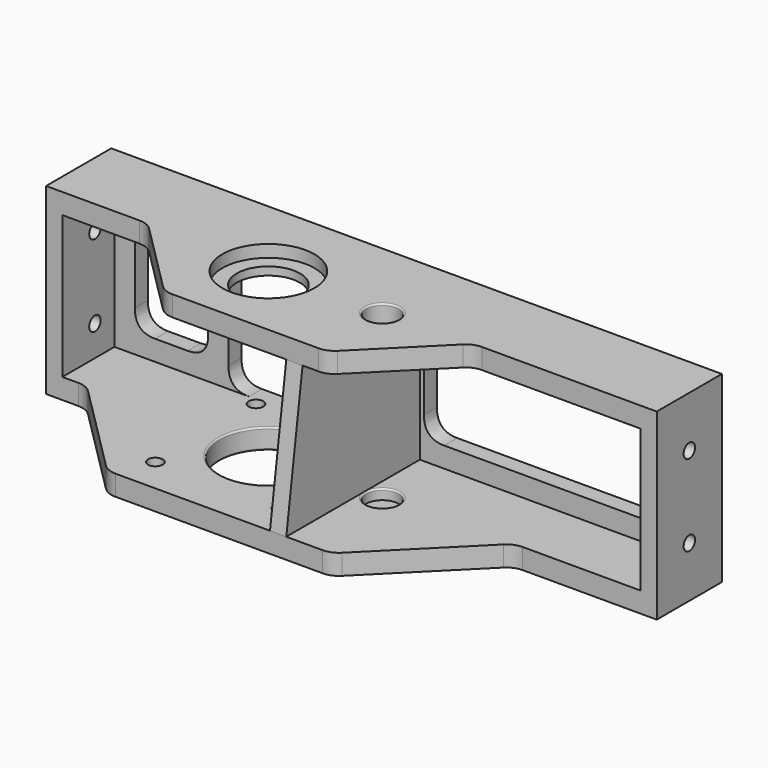
from build123d import *

# Parameters (mm, degrees)
F0_R         = 1.8
F0_R_2       = 12
F0_R_3       = 4
F1_DEPTH     = 5
F2_W         = 4
F2_H         = 20
F3_DEPTH     = 40
F4_R         = 12.5
F4_R_2       = 11.3
F4_R_3       = 7.75
F5_DEPTH     = 5
F6_DEPTH     = 50
F7_DEPTH     = 3
F8_R         = 5
F9_R         = 0.4
F10_DEPTH    = 2.5
F11_R        = 1.75
F12_DEPTH    = 150.001
F13_W        = 28
F13_H        = 4
F13_W_2      = 71
F14_DEPTH    = 40
F15_W        = 18
F15_H        = 25
F15_W_2      = 61
F16_DEPTH    = 25
F17_T1_DEPTH = 4
F19_DEPTH    = 41
F21_DEPTH    = 5


# Not quite as in the source:
# - a fillet or chamfer that OpenCascade refuses, or shapes differently, is made with other operations: its cross-section is extruded or revolved along the edge and cut away or added


with BuildPart() as f1:
    # F0 (on Top) → F1 (new body)
    with BuildSketch(Plane.XY):
        Polygon((75, 27), (-75, 27), (-75, 7), (-65, 7), (-40, -18), (15, -18), (40, 7), (75, 7), align=None)
        with Locations((-35, -9.44)):
            Circle(F0_R, mode=Mode.SUBTRACT)
        with Locations((-4.2, -9.44)):
            Circle(F0_R, mode=Mode.SUBTRACT)
        with Locations((-19.6, 6)):
            Circle(F0_R_2, mode=Mode.SUBTRACT)
        with Locations((-35, 21.44)):
            Circle(F0_R, mode=Mode.SUBTRACT)
        with Locations((-4.2, 21.44)):
            Circle(F0_R, mode=Mode.SUBTRACT)
        with Locations((8.4, 6)):
            Circle(F0_R_3, mode=Mode.SUBTRACT)
    extrude(amount=F1_DEPTH)

    # F2 (on face) → F3 (join)
    with BuildSketch(Plane.XY.offset(5)):
        with Locations((-73, 17)):
            Rectangle(F2_W, F2_H)
        with Locations((73, 17)):
            Rectangle(F2_W, F2_H)
    extrude(amount=F3_DEPTH)

    # F4 (on face) → F5 (join)
    with BuildSketch(Plane.XY.offset(45)):
        Polygon((71, 7), (71, 27), (-75, 27), (-75, 7), (-50, 7), (-30, -13), (10, -13), (30, 7), align=None)
        with Locations((-19.6, 6)):
            Circle(F4_R, mode=Mode.SUBTRACT)
        with Locations((-19.6, 6)):
            Circle(F4_R)
        with Locations((-19.6, 6)):
            Circle(F4_R_2, mode=Mode.SUBTRACT)
        with Locations((-19.6, 6)):
            Circle(F4_R_2)
        with Locations((-19.6, 6)):
            Circle(F4_R_3, mode=Mode.SUBTRACT)
    extrude(amount=-F5_DEPTH)

    # F0 (on Top) → F6 (cut)
    with BuildSketch(Plane.XY):
        with Locations((8.4, 6)):
            Circle(F0_R_3)
    extrude(amount=F6_DEPTH, mode=Mode.SUBTRACT)

    # F4 (on face) → F7 (cut)
    with BuildSketch(Plane.XY.offset(45)):
        with Locations((-19.6, 6)):
            Circle(F4_R_2)
        with Locations((-19.6, 6)):
            Circle(F4_R_3, mode=Mode.SUBTRACT)
    extrude(amount=-F7_DEPTH, mode=Mode.SUBTRACT)

    # F8
    f8_edges = [f1.edges().sort_by_distance(p)[0] for p in [
        (-65, 7, 2.5),
        (-40, -18, 2.5),
        (40, 7, 2.5),
        (15, -18, 2.5),
        (-50, 7, 42.5),
        (-30, -13, 42.5),
        (10, -13, 42.5),
        (30, 7, 42.5),
    ]]
    fillet(f8_edges, radius=F8_R)

    # F9
    f9_edges = [f1.edges().sort_by_distance(p)[0] for p in [
        (-31.6, 6, 5),
        (-31.6, 6, 0),
        (4.4, 6, 5),
        (4.4, 6, 45),
        (4.4, 6, 40),
    ]]
    fillet(f9_edges, radius=F9_R)

    # F0 (on Top) → F10 (join)
    with BuildSketch(Plane.XY):
        with Locations((8.4, 6)):
            Circle(F0_R_3)
    extrude(amount=F10_DEPTH)

    # F11 (on face) → F12 (cut, through all)
    with BuildSketch(Plane.YZ.offset(75)):
        with Locations((17, 32.5)):
            Circle(F11_R)
        with Locations((17, 12.5)):
            Circle(F11_R)
    extrude(amount=-F12_DEPTH, mode=Mode.SUBTRACT)

    # F13 (on face) → F14 (join)
    with BuildSketch(Plane.XY.offset(5)):
        with Locations((-57, 25)):
            Rectangle(F13_W, F13_H)
        with Locations((35.5, 25)):
            Rectangle(F13_W_2, F13_H)
    extrude(amount=F14_DEPTH)

    # F15 (on face) → F16 (cut)
    with BuildSketch(Plane.XZ.offset(-23)):
        with Locations((-57, 22.5)):
            Rectangle(F15_W, F15_H)
        with Locations((35.5, 22.5)):
            Rectangle(F15_W_2, F15_H)
    extrude(amount=-F16_DEPTH, mode=Mode.SUBTRACT)

    # F17: fillet of radius 5 on 11 edges, made by hand

    # F17_s2 → F17_t1 (join)
    with BuildSketch(Plane.XZ.offset(-27)):
        with BuildLine():
            add(Edge.make_bspline(
                [(-61, 35), (-66, 35), (-66, 30)],
                knots=[0, 0, 0, 1, 1, 1], degree=2, weights=[1, 1, 1]))
            Line((-66, 30), (-66, 35))
            Line((-66, 35), (-61, 35))
        make_face()
        with BuildLine():
            add(Edge.make_bspline(
                [(10, 35), (5, 35), (5, 30)],
                knots=[0, 0, 0, 1, 1, 1], degree=2, weights=[1, 1, 1]))
            Line((5, 30), (5, 35))
            Line((5, 35), (10, 35))
        make_face()
        with BuildLine():
            add(Edge.make_bspline(
                [(-53, 10), (-48, 10), (-48, 15)],
                knots=[0, 0, 0, 1, 1, 1], degree=2, weights=[1, 1, 1]))
            Line((-48, 15), (-48, 10))
            Line((-48, 10), (-53, 10))
        make_face()
        with BuildLine():
            add(Edge.make_bspline(
                [(61, 10), (66, 10), (66, 15)],
                knots=[0, 0, 0, 1, 1, 1], degree=2, weights=[1, 1, 1]))
            Line((66, 15), (66, 10))
            Line((66, 10), (61, 10))
        make_face()
        with BuildLine():
            add(Edge.make_bspline(
                [(61, 35), (66, 35), (66, 30)],
                knots=[0, 0, 0, 1, 1, 1], degree=2, weights=[1, 1, 1]))
            Line((66, 30), (66, 35))
            Line((66, 35), (61, 35))
        make_face()
        with BuildLine():
            add(Edge.make_bspline(
                [(-5, 40), (0, 40), (0, 35)],
                knots=[0, 0, 0, 1, 1, 1], degree=2, weights=[1, 1, 1]))
            Line((0, 35), (0, 40))
            Line((0, 40), (-5, 40))
        make_face()
        with BuildLine():
            add(Edge.make_bspline(
                [(-53, 35), (-48, 35), (-48, 30)],
                knots=[0, 0, 0, 1, 1, 1], degree=2, weights=[1, 1, 1]))
            Line((-48, 30), (-48, 35))
            Line((-48, 35), (-53, 35))
        make_face()
        with BuildLine():
            add(Edge.make_bspline(
                [(-38, 5), (-43, 5), (-43, 10)],
                knots=[0, 0, 0, 1, 1, 1], degree=2, weights=[1, 1, 1]))
            Line((-43, 10), (-43, 5))
            Line((-43, 5), (-38, 5))
        make_face()
        with BuildLine():
            add(Edge.make_bspline(
                [(-66, 15), (-66, 10), (-61, 10)],
                knots=[0, 0, 0, 1, 1, 1], degree=2, weights=[1, 1, 1]))
            Line((-61, 10), (-66, 10))
            Line((-66, 10), (-66, 15))
        make_face()
        with BuildLine():
            add(Edge.make_bspline(
                [(5, 15), (5, 10), (10, 10)],
                knots=[0, 0, 0, 1, 1, 1], degree=2, weights=[1, 1, 1]))
            Line((10, 10), (5, 10))
            Line((5, 10), (5, 15))
        make_face()
        with BuildLine():
            add(Edge.make_bspline(
                [(-38, 40), (-43, 40), (-43, 35)],
                knots=[0, 0, 0, 1, 1, 1], degree=2, weights=[1, 1, 1]))
            Line((-43, 35), (-43, 40))
            Line((-43, 40), (-38, 40))
        make_face()
    extrude(amount=F17_T1_DEPTH)

    # F18 (on face) → F19 (join)
    with BuildSketch(Plane.XZ.offset(-23)):
        Polygon((0, 35), (0, 5), (3.9987709172, 5), (3.9987709172, 40), (0, 40), align=None)
    extrude(amount=F19_DEPTH)

    # F20 (on face) → F21 (cut)
    with BuildSketch(Plane.YZ.offset(3.9987709172)):
        Polygon((-18, 5), (-13, 40), (-18, 40), align=None)
    extrude(amount=-F21_DEPTH, mode=Mode.SUBTRACT)


solid = f1.part
